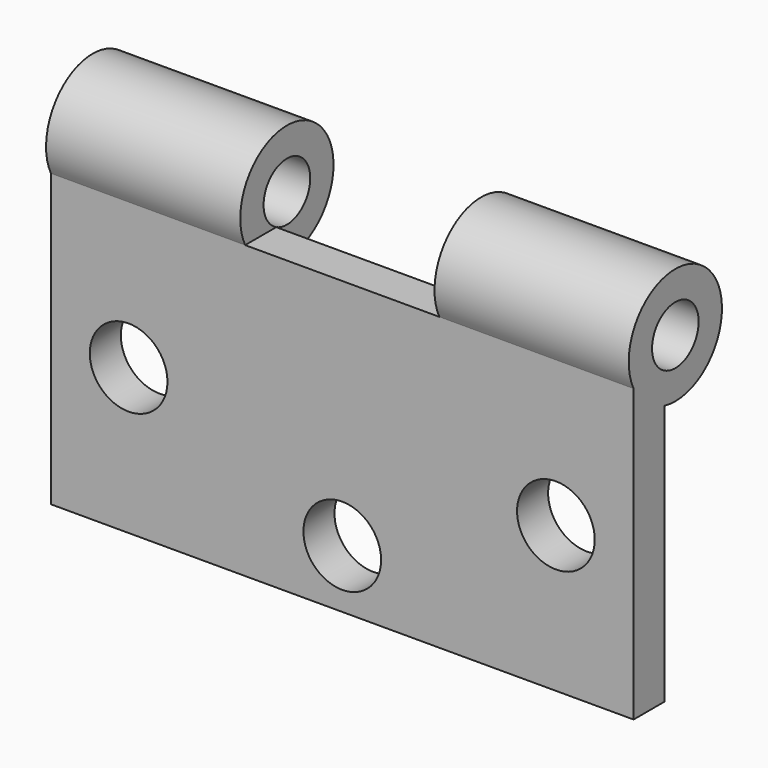
from build123d import *

# Parameters (mm, degrees)
F0_W     = 76.2
F0_H     = 38.1
F1_DEPTH = 5.08
F2_R     = 7.62
F2_R_2   = 3.81
F3_DEPTH = 25.4
F4_R     = 7.62
F4_R_2   = 3.81
F5_DEPTH = 25.4
F6_R     = 5.08
F7_DEPTH = 5.08


# Not quite as in the source:
# - a feature names something its author has since deleted; it is built from what else it names


with BuildPart() as f1:
    # F0 (on Front) → F1 (new body)
    with BuildSketch(Plane.XZ):
        with Locations((-22.0833101058, -12.6055886477)):
            Rectangle(F0_W, F0_H)
    extrude(amount=F1_DEPTH)

    # F2 (on face) → F3 (join)
    with BuildSketch(Plane.YZ.offset(16.0166898942)):
        with Locations((1.74625, 9.8306645822)):
            Circle(F2_R)
        with Locations((1.74625, 9.8306645822)):
            Circle(F2_R_2, mode=Mode.SUBTRACT)
    extrude(amount=-F3_DEPTH)

    # F4 (on face) → F5 (join)
    with BuildSketch(Plane(origin=(-60.1833101058, 0, 0), x_dir=(0, -1, 0), z_dir=(-1, 0, 0))):
        with Locations((-1.74625, 9.8306645822)):
            Circle(F4_R)
        with Locations((-1.74625, 9.8306645822)):
            Circle(F4_R_2, mode=Mode.SUBTRACT)
    extrude(amount=-F5_DEPTH)

    # F6 (on face) → F7 (cut, through all)
    with BuildSketch(Plane.XZ.offset(5.08)):
        with Locations((-50.0233101058, -12.6055886477)):
            Circle(F6_R)
        with Locations((-22.0833101058, -24.0355886477)):
            Circle(F6_R)
        with Locations((5.8566898942, -12.6055886477)):
            Circle(F6_R)
    extrude(amount=-F7_DEPTH, mode=Mode.SUBTRACT)


solid = f1.part
